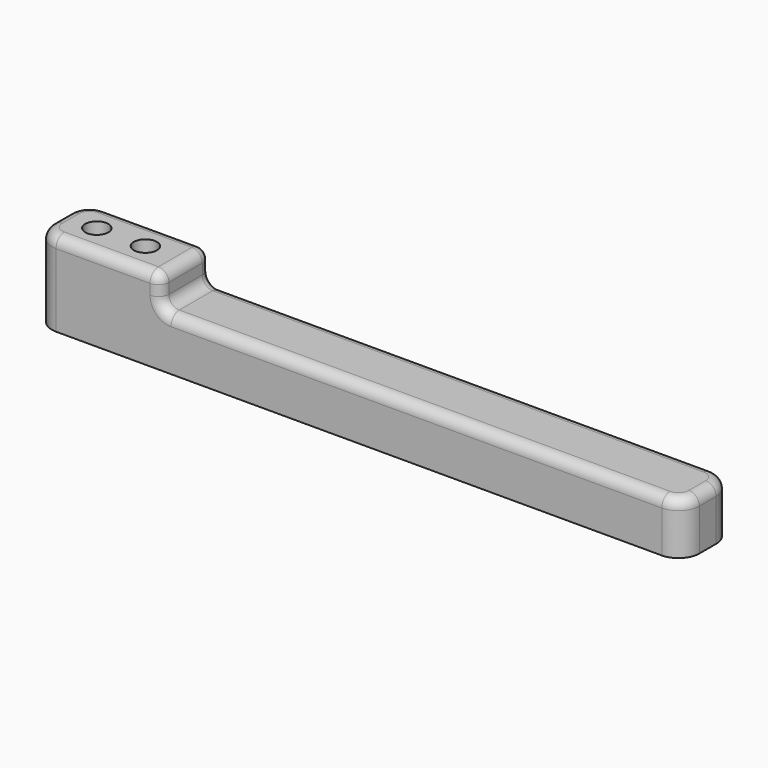
from build123d import *

# Parameters (mm, degrees)
F0_W         = 12
F0_H         = 6
F0_R         = 1.1
F1_DEPTH     = 8
F3_DEPTH     = 5
F4_SIZE      = 0.5
F5_F1_R      = 1
F5_F2_R      = 1
F6_T1_DEPTH  = 13
F6_T3_DEPTH  = 10
F6_T6_ANGLE  = 90
F6_T8_ANGLE  = 90
F6_T10_ANGLE = 90
F6_T12_ANGLE = 90


# Not quite as in the source:
# - a fillet or chamfer that OpenCascade refuses, or shapes differently, is made with other operations: its cross-section is extruded or revolved along the edge and cut away or added


with BuildPart() as f1:
    # F0 (on Top) → F1 (new body)
    with BuildSketch(Plane.XY):
        Rectangle(F0_W, F0_H)
        with Locations((-2.5, 0)):
            Circle(F0_R, mode=Mode.SUBTRACT)
        with BuildLine():
            ThreePointArc((1.05, 0), (2.15, 1.1), (3.25, 0))
            ThreePointArc((3.25, 0), (2.15, -1.1), (1.05, 0))
        make_face(mode=Mode.SUBTRACT)
    extrude(amount=F1_DEPTH)

    # F2 (on Top) → F3 (join)
    with BuildSketch(Plane.XY):
        Polygon((56, -3), (56, 0), (56, 3), (6, 3), (6, 0), (6, -3), align=None)
    extrude(amount=F3_DEPTH)

    # F4
    f4_edges = [f1.edges().sort_by_distance(p)[0] for p in [
        (-3.6, 0, 0),
        (1.05, 0, 0),
    ]]
    chamfer(f4_edges, length=F4_SIZE)

    # F5: fillet of radius 1 on 8 edges, made by hand

    # F5_f1
    f5_f1_edges = [f1.edges().sort_by_distance(p)[0] for p in [
        (6, 0, 5),
    ]]
    fillet(f5_f1_edges, radius=F5_F1_R)

    # F5_f2
    f5_f2_edges = [f1.edges().sort_by_distance(p)[0] for p in [
        (6, -3, 7),
        (6, 3, 7),
        (56, 0, 5),
        (0, -3, 8),
        (6, 0, 8),
        (0, 3, 8),
        (-6, 0, 8),
        (6.2928932188, 3, 5.2928932188),
        (6.2928932188, -3, 5.2928932188),
    ]]
    fillet(f5_f2_edges, radius=F5_F2_R)

    # F6: fillet of radius 2 on 4 edges, made by hand

    # F6_s2 → F6_t1 (cut)
    with BuildSketch(Plane.XY.offset(-5)):
        with BuildLine():
            ThreePointArc((-4, -3), (-5.4142135624, -2.4142135624), (-6, -1))
            Line((-6, -1), (-6, -3))
            Line((-6, -3), (-4, -3))
        make_face()
        with BuildLine():
            ThreePointArc((-6, 1), (-5.4142135624, 2.4142135624), (-4, 3))
            Line((-4, 3), (-6, 3))
            Line((-6, 3), (-6, 1))
        make_face()
    extrude(amount=F6_T1_DEPTH, mode=Mode.SUBTRACT)

    # F6_s4 → F6_t3 (cut)
    with BuildSketch(Plane.XY.offset(-5)):
        with BuildLine():
            ThreePointArc((54, -3), (55.4142135624, -2.4142135624), (56, -1))
            Line((56, -1), (56, -3))
            Line((56, -3), (54, -3))
        make_face()
        with BuildLine():
            ThreePointArc((56, 1), (55.4142135624, 2.4142135624), (54, 3))
            Line((54, 3), (56, 3))
            Line((56, 3), (56, 1))
        make_face()
    extrude(amount=F6_T3_DEPTH, mode=Mode.SUBTRACT)

    # F6_s5 → F6_t6 (revolve, cut)
    with BuildSketch(Plane.XZ.offset(-1)):
        with BuildLine():
            ThreePointArc((55, 5), (55.7071067812, 4.7071067812), (56, 4))
            Line((56, 4), (56, 5))
            Line((56, 5), (55, 5))
        make_face()
    revolve(axis=Axis((54, 1, 5), (0, 0, 1)), revolution_arc=F6_T6_ANGLE, mode=Mode.SUBTRACT)

    # F6_s7 → F6_t8 (revolve, cut)
    with BuildSketch(Plane.YZ.offset(54)):
        with BuildLine():
            ThreePointArc((-2, 5), (-2.7071067812, 4.7071067812), (-3, 4))
            Line((-3, 4), (-3, 5))
            Line((-3, 5), (-2, 5))
        make_face()
    revolve(axis=Axis((54, -1, 5), (0, 0, 1)), revolution_arc=F6_T8_ANGLE, mode=Mode.SUBTRACT)

    # F6_s9 → F6_t10 (revolve, cut)
    with BuildSketch(Plane.YZ.offset(-4)):
        with BuildLine():
            ThreePointArc((2, 8), (2.7071067812, 7.7071067812), (3, 7))
            Line((3, 7), (3, 8))
            Line((3, 8), (2, 8))
        make_face()
    revolve(axis=Axis((-4, 1, 8), (0, 0, 1)), revolution_arc=F6_T10_ANGLE, mode=Mode.SUBTRACT)

    # F6_s11 → F6_t12 (revolve, cut)
    with BuildSketch(Plane.XZ.offset(1)):
        with BuildLine():
            ThreePointArc((-5, 8), (-5.7071067812, 7.7071067812), (-6, 7))
            Line((-6, 7), (-6, 8))
            Line((-6, 8), (-5, 8))
        make_face()
    revolve(axis=Axis((-4, -1, 8), (0, 0, 1)), revolution_arc=F6_T12_ANGLE, mode=Mode.SUBTRACT)


solid = f1.part
